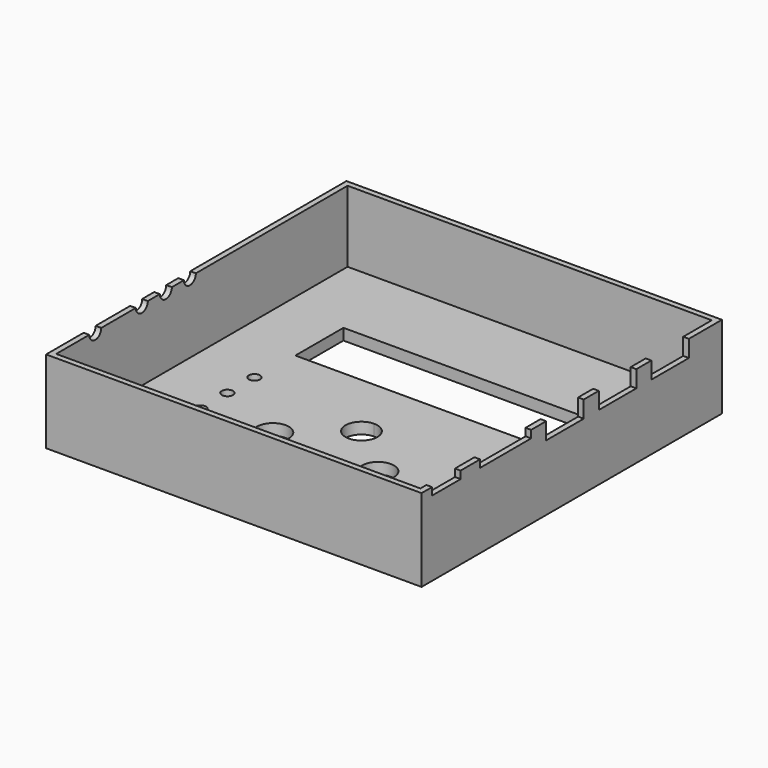
from build123d import *

# Parameters (mm, degrees)
F0_R      = 1.5
F0_R_2    = 4.25
F1_DEPTH  = 3
F2_DEPTH  = 22
F3_W      = 9.5
F3_H      = 11
F2_FACE_W = 100
F2_FACE_H = 22
F4_DEPTH  = 50.001
F5_W      = 17
F5_H      = 3.3289747284
F6_DEPTH  = 76.9
F7_W      = 12.5
F7_H      = 8.2103219628
F7_H_2    = 8.3398447186
F7_H_3    = 8.5524427253
F8_DEPTH  = 63.2
F9_R      = 2
F10_DEPTH = 67.3


# Not quite as in the source:
# - a feature of the source that left no trace in its solid (it failed there, or was rolled back) is left out


with BuildPart() as f1:
    # F0 (on Top) → F1 (new body)
    with BuildSketch(Plane.XY):
        with BuildLine():
            Line((-48.5, -48.5), (0, -48.5))
            Line((0, -48.5), (0, -35.75))
            ThreePointArc((0, -35.75), (-4.25, -31.5), (0, -27.25))
            Line((0, -27.25), (0, -11.75))
            ThreePointArc((0, -11.75), (-4.25, -7.5), (0, -3.25))
            Line((0, -3.25), (0, 10.5))
            Line((0, 10.5), (-32, 10.5))
            Line((-32, 10.5), (-32, 26.5))
            Line((-32, 26.5), (0, 26.5))
            Line((0, 26.5), (0, 48.5))
            Line((0, 48.5), (-48.5, 48.5))
            Line((-48.5, 48.5), (-48.5, -48.5))
        make_face()
        with Locations((-32.5, -20.5)):
            Circle(F0_R, mode=Mode.SUBTRACT)
        with Locations((-32.5, -11.5)):
            Circle(F0_R, mode=Mode.SUBTRACT)
        with Locations((-32.5, -2.5)):
            Circle(F0_R, mode=Mode.SUBTRACT)
        with Locations((-14, -19.5)):
            Circle(F0_R_2, mode=Mode.SUBTRACT)
        with BuildLine():
            Line((0, -35.75), (0, -48.5))
            Line((0, -48.5), (48.5, -48.5))
            Line((48.5, -48.5), (48.5, 48.5))
            Line((48.5, 48.5), (0, 48.5))
            Line((0, 48.5), (0, 26.5))
            Line((0, 26.5), (32, 26.5))
            Line((32, 26.5), (32, 10.5))
            Line((32, 10.5), (0, 10.5))
            Line((0, 10.5), (0, -3.25))
            ThreePointArc((0, -3.25), (3.00520382, -4.49479618), (4.25, -7.5))
            ThreePointArc((4.25, -7.5), (3.00520382, -10.50520382), (0, -11.75))
            Line((0, -11.75), (0, -27.25))
            ThreePointArc((0, -27.25), (3.00520382, -28.49479618), (4.25, -31.5))
            ThreePointArc((4.25, -31.5), (3.00520382, -34.50520382), (0, -35.75))
        make_face()
        with Locations((14, -19.5)):
            Circle(F0_R_2, mode=Mode.SUBTRACT)
    extrude(amount=F1_DEPTH)

    # F0 (on Top) → F2 (join)
    with BuildSketch(Plane.XY):
        Polygon((50, 50), (-50, 50), (-50, -50), (0, -50), (50, -50), align=None)
        Polygon((48.5, -48.5), (0, -48.5), (-48.5, -48.5), (-48.5, 48.5), (0, 48.5), (48.5, 48.5), align=None, mode=Mode.SUBTRACT)
    extrude(amount=F2_DEPTH)

    # F3 (on Right) + F2_face (on face) → F4 (cut, through all)
    with BuildSketch(Plane.YZ):
        with Locations((-41.75, 25.5)):
            Rectangle(F3_W, F3_H)
    with BuildSketch(Plane(origin=(50, 0, 11), x_dir=(0, 1, 0), z_dir=(1, 0, 0))):
        Rectangle(F2_FACE_W, F2_FACE_H)
    extrude(amount=F4_DEPTH, mode=Mode.SUBTRACT)

    # F5 (on Right) → F6 (cut)
    with BuildSketch(Plane.YZ):
        with Locations((-22, 21.6644873642)):
            Rectangle(F5_W, F5_H)
    extrude(amount=F6_DEPTH, mode=Mode.SUBTRACT)

    # F7 (on Right) → F8 (cut)
    with BuildSketch(Plane.YZ):
        with Locations((32.75, 21.6051609814)):
            Rectangle(F7_W, F7_H)
        with Locations((15.25, 21.6699223593)):
            Rectangle(F7_W, F7_H_2)
        with Locations((-2.25, 21.7762213627)):
            Rectangle(F7_W, F7_H_3)
    extrude(amount=F8_DEPTH, mode=Mode.SUBTRACT)

    # F9 (on Right) → F10 (cut)
    with BuildSketch(Plane.YZ):
        with Locations((-12, 22)):
            Circle(F9_R)
        with Locations((-4, 22)):
            Circle(F9_R)
        with Locations((-20, 22)):
            Circle(F9_R)
        with Locations((-35.5, 22)):
            Circle(F9_R)
    extrude(amount=-F10_DEPTH, mode=Mode.SUBTRACT)


solid = f1.part
